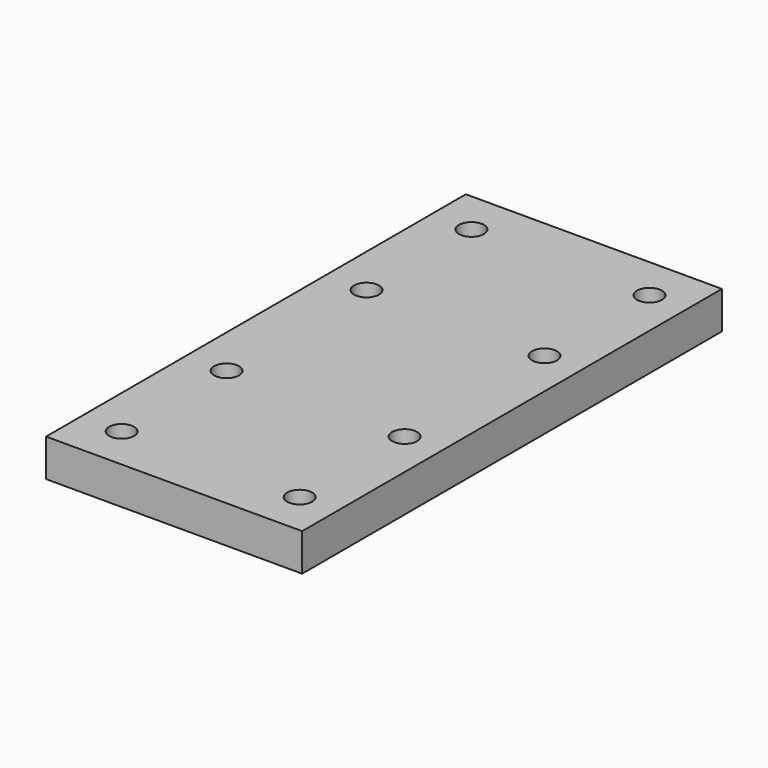
from build123d import *

# Parameters (mm, degrees)
F0_W     = 41
F0_H     = 84
F1_DEPTH = 6
F3_R     = 2
F4_DEPTH = 6


# Not quite as in the source:
# - a feature names something its author has since deleted; it is built from what else it names


with BuildPart() as f1:
    # F0 (on Top) → F1 (new body)
    with BuildSketch(Plane.XY):
        Rectangle(F0_W, F0_H)
    extrude(amount=F1_DEPTH)

    # F3 (on face) → F4 (cut, through all)
    with BuildSketch(Plane.XY.offset(6)):
        with Locations((-14, 14)):
            Circle(F3_R)
        with Locations((-14, -14)):
            Circle(F3_R)
        with Locations((14.5, 14)):
            Circle(F3_R)
        with Locations((14.5, -14)):
            Circle(F3_R)
        with Locations((14.5, -35)):
            Circle(F3_R)
        with Locations((14.5, 35)):
            Circle(F3_R)
        with Locations((-14, 35)):
            Circle(F3_R)
        with Locations((-14, -35)):
            Circle(F3_R)
    extrude(amount=-F4_DEPTH, mode=Mode.SUBTRACT)


solid = f1.part
